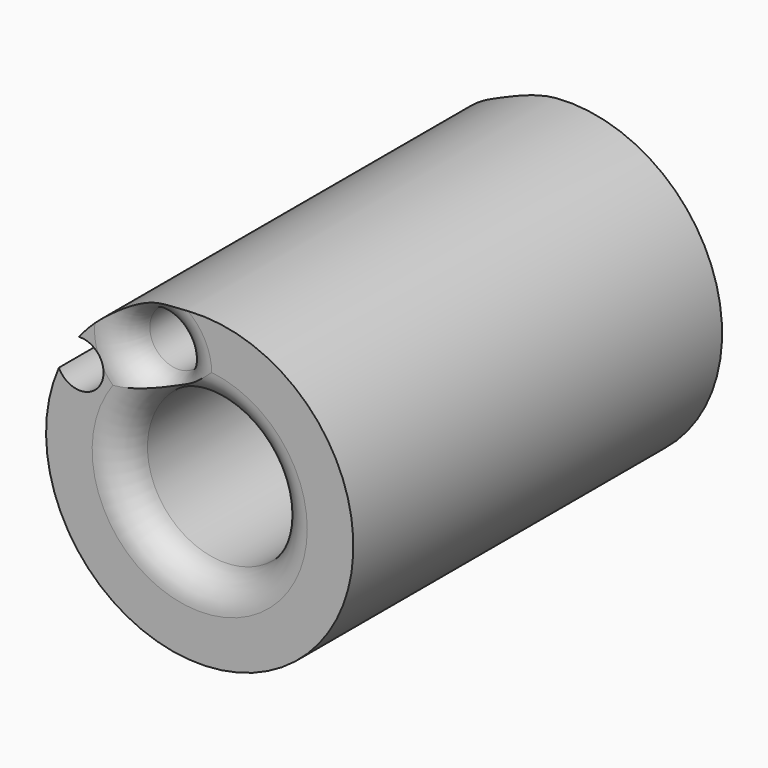
from build123d import *

# Parameters (mm, degrees)
F0_R     = 25.4
F1_DEPTH = 76.2
F2_R     = 12.7
F3_DEPTH = 105.41
F4_R     = 3.8838784961
F5_DEPTH = 133.35
F6_R     = 4.6082025667
F7_DEPTH = 145.542


# Not quite as in the source:
# - a fillet or chamfer that OpenCascade refuses, or shapes differently, is made with other operations: its cross-section is extruded or revolved along the edge and cut away or added


with BuildPart() as f1:
    # F0 (on Front) → F1 (new body)
    with BuildSketch(Plane.XZ):
        Circle(F0_R)
    extrude(amount=F1_DEPTH)

    # F2 (on face) → F3 (cut)
    with BuildSketch(Plane.XZ.offset(76.2)):
        Circle(F2_R)
    extrude(amount=-F3_DEPTH, mode=Mode.SUBTRACT)

    # F4 (on Front) → F5 (cut)
    with BuildSketch(Plane.XZ):
        with Locations((-19.7816453874, 11.8296807632)):
            Circle(F4_R)
    extrude(amount=F5_DEPTH, mode=Mode.SUBTRACT)

    # F6 (on Front) → F7 (cut)
    with BuildSketch(Plane.XZ):
        with Locations((-7.7014984563, 17.5422988832)):
            Circle(F6_R)
    extrude(amount=F7_DEPTH, mode=Mode.SUBTRACT)

    # F8: fillet of radius 5.08 on 2 edges, made by hand

    # F8_s1 → F8_t2 (revolve, cut)
    with BuildSketch(Plane.XY):
        with BuildLine():
            ThreePointArc((17.78, -76.2), (14.1878975516, -74.7121024484), (12.7, -71.12))
            Line((12.7, -71.12), (12.7, -76.2))
            Line((12.7, -76.2), (17.78, -76.2))
        make_face()
    revolve(axis=Axis((0, -76.2, 0), (0, -1, 0)), mode=Mode.SUBTRACT)

    # F8_s3 → F8_t4 (revolve, cut)
    with BuildSketch(Plane.XY.offset(17.5422988832)):
        with BuildLine():
            ThreePointArc((1.9867041104, -76.2), (-1.605398338, -74.7121024484), (-3.0932958896, -71.12))
            Line((-3.0932958896, -71.12), (-3.0932958896, -76.2))
            Line((-3.0932958896, -76.2), (1.9867041104, -76.2))
        make_face()
    revolve(axis=Axis((-7.7014984563, -76.2, 17.5422988832), (0, 1, 0)), mode=Mode.SUBTRACT)

    # F9: fillet of radius 5.08 on 2 edges, made by hand

    # F9_s1 → F9_t2 (revolve, cut)
    with BuildSketch(Plane.XY):
        with BuildLine():
            ThreePointArc((17.7809656854, 0.0004), (14.1878975516, -1.4878975516), (12.6996, -5.0809656854))
            Line((12.6996, -5.0809656854), (12.1914634315, -5.0809656854))
            ThreePointArc((12.1914634315, -5.0809656854), (12.1918634315, -2.5404828427), (12.1918634315, 0))
            Line((12.1918634315, 0), (12.7, 0.5081365685))
            ThreePointArc((12.7, 0.5081365685), (15.2404828427, 0.5081365685), (17.7809656854, 0.5085365685))
            Line((17.7809656854, 0.5085365685), (17.7809656854, 0.0004))
        make_face()
    revolve(axis=Axis((0, 0, 0), (0, -1, 0)), mode=Mode.SUBTRACT)

    # F9_s3 → F9_t4 (revolve, cut)
    with BuildSketch(Plane.XY.offset(17.5422988832)):
        with BuildLine():
            ThreePointArc((1.9876697958, 0.0004), (-1.605398338, -1.4878975516), (-3.0936958896, -5.0809656854))
            Line((-3.0936958896, -5.0809656854), (-3.6018324581, -5.0809656854))
            ThreePointArc((-3.6018324581, -5.0809656854), (-3.6014324581, -2.5404828427), (-3.6014324581, 0))
            Line((-3.6014324581, 0), (-3.0932958896, 0.5081365685))
            ThreePointArc((-3.0932958896, 0.5081365685), (-0.5528130469, 0.5081365685), (1.9876697958, 0.5085365685))
            Line((1.9876697958, 0.5085365685), (1.9876697958, 0.0004))
        make_face()
    revolve(axis=Axis((-7.7014984563, 0, 17.5422988832), (0, -1, 0)), mode=Mode.SUBTRACT)


solid = f1.part
